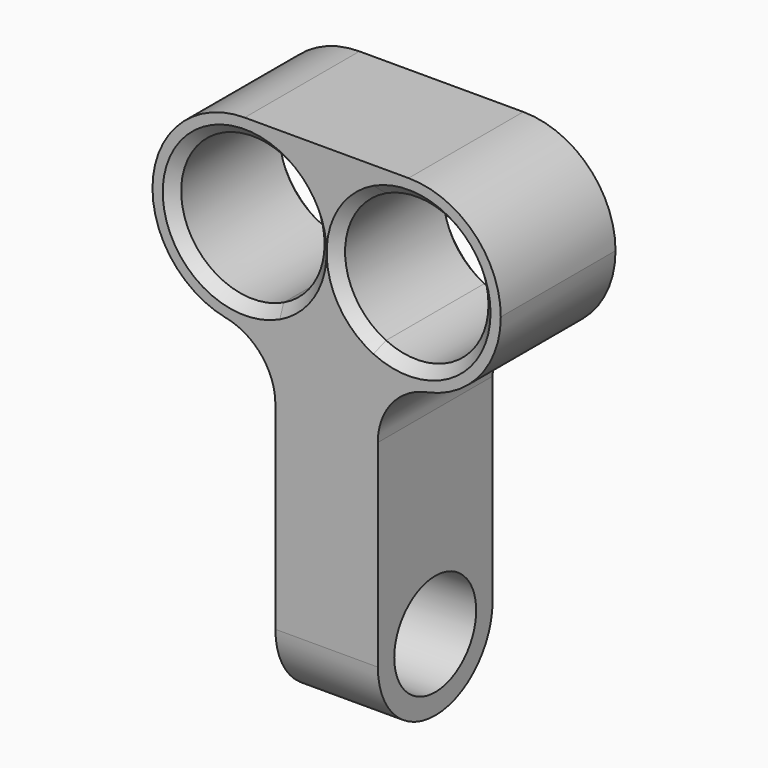
from build123d import *

# Parameters (mm, degrees)
F0_W     = 5
F0_H     = 16
F1_DEPTH = 7
F3_D     = 5
F4_R     = 4.49999
F5_R     = 3.49999
F6_R     = 3
F7_SIZE  = 0.49999


# Not quite as in the source:
# - a fillet or chamfer is up to 0.001 mm smaller than in the source, because OpenCascade refuses the exact size


with BuildPart() as f1:
    # F0 (on Front) → F1 (new body)
    with BuildSketch(Plane.XZ):
        with BuildLine():
            Line((8.5, 12.5), (2.5, 12.5))
            Line((2.5, 12.5), (2.5, 11.1622776602))
            ThreePointArc((2.5, 11.1622776602), (5.8708286934, 10.9580398915), (7.5, 8))
            ThreePointArc((7.5, 8), (5.8708286934, 5.0419601085), (2.5, 4.8377223398))
            Line((2.5, 4.8377223398), (2.5, 3.5))
            Line((2.5, 3.5), (8.5, 3.5))
            Line((8.5, 3.5), (8.5, 12.5))
        make_face()
        with BuildLine():
            Line((-2.5, 11.1622776602), (-2.5, 12.5))
            Line((-2.5, 12.5), (-8.5, 12.5))
            Line((-8.5, 12.5), (-8.5, 3.5))
            Line((-8.5, 3.5), (-2.5, 3.5))
            Line((-2.5, 3.5), (-2.5, 4.8377223398))
            ThreePointArc((-2.5, 4.8377223398), (-7.5, 8), (-2.5, 11.1622776602))
        make_face()
        with BuildLine():
            Line((2.5, 11.1622776602), (2.5, 12.5))
            Line((2.5, 12.5), (-2.5, 12.5))
            Line((-2.5, 12.5), (-2.5, 11.1622776602))
            ThreePointArc((-2.5, 11.1622776602), (-1.0419601085, 9.8708286934), (-0.5, 8))
            ThreePointArc((-0.5, 8), (-1.0419601085, 6.1291713066), (-2.5, 4.8377223398))
            Line((-2.5, 4.8377223398), (-2.5, 3.5))
            Line((-2.5, 3.5), (2.5, 3.5))
            Line((2.5, 3.5), (2.5, 4.8377223398))
            ThreePointArc((2.5, 4.8377223398), (0.5, 8), (2.5, 11.1622776602))
        make_face()
        with Locations((0, -4.5)):
            Rectangle(F0_W, F0_H)
    extrude(amount=F1_DEPTH)

    # F3 (through all)
    with Locations(Plane.YZ.offset(2.5)):
        with Locations((-3.5, -9)):
            Hole(F3_D / 2)

    # F4 (radius 4.5 in the source; OpenCascade refuses exactly that, so slightly less here)
    f4_edges = [f1.edges().sort_by_distance(p)[0] for p in [
        (8.5, -3.5, 12.5),
        (-8.5, -3.5, 12.5),
        (8.5, -3.5, 3.5),
        (-8.5, -3.5, 3.5),
    ]]
    fillet(f4_edges, radius=F4_R)

    # F5 (radius 3.5 in the source; OpenCascade refuses exactly that, so slightly less here)
    f5_edges = [f1.edges().sort_by_distance(p)[0] for p in [
        (0, 0, -12.5),
        (0, -7, -12.5),
    ]]
    fillet(f5_edges, radius=F5_R)

    # F6
    f6_edges = [f1.edges().sort_by_distance(p)[0] for p in [
        (2.5, -3.5, 3.5),
        (-2.5, -3.5, 3.5),
    ]]
    fillet(f6_edges, radius=F6_R)

    # F7 (size 0.5 in the source; OpenCascade refuses exactly that, so slightly less here)
    f7_edges = [f1.edges().sort_by_distance(p)[0] for p in [
        (-7.5, -7, 8),
        (5.5, -7, 11.162278),
        (-7.5, 0, 8),
        (5.5, 0, 11.162278),
    ]]
    chamfer(f7_edges, length=F7_SIZE)


solid = f1.part
